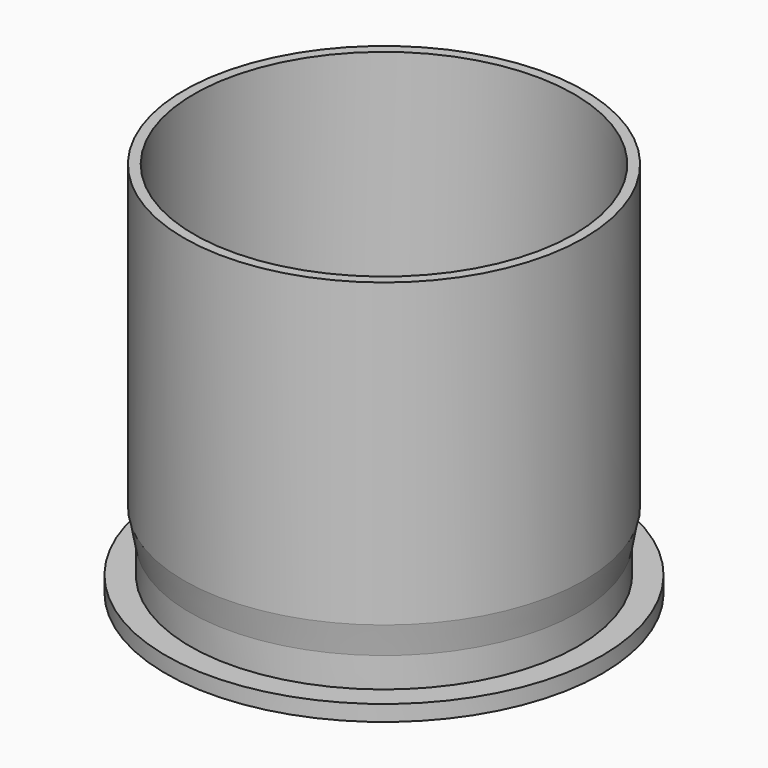
from build123d import *

# Parameters (mm, degrees)
F0_R     = 21.8313
F1_DEPTH = 1.5875
F2_R     = 19.3793862589
F3_DEPTH = 3
F4_R     = 19.4142729727
F5_DEPTH = 3
F5_TAPER = -10
F6_R     = 20
F7_DEPTH = 30.1498
F8_T     = 1
F10_D    = 12.7


# Not quite as in the source:
# - a length typed as a fraction of an inch, garbled in the dataset ("3 / 203.2 mm" for 3/8 in), is restored
# - a shell that OpenCascade refuses in one call is made with other operations: the cavity is built on its own and cut out


with BuildPart() as f1:
    # F0 (on Top) → F1 (new body)
    with BuildSketch(Plane.XY):
        Circle(F0_R)
    extrude(amount=F1_DEPTH)

    # F2 (on face) → F3 (join)
    with BuildSketch(Plane.XY.offset(1.5875)):
        Circle(F2_R)
    extrude(amount=F3_DEPTH)

    # F4 (on face) → F5 (join)
    with BuildSketch(Plane.XY.offset(4.5875)):
        Circle(F4_R)
    extrude(amount=F5_DEPTH, taper=F5_TAPER)

    # F6 (on face) → F7 (join)
    with BuildSketch(Plane.XY.offset(7.5875)):
        Circle(F6_R)
    extrude(amount=F7_DEPTH)

    # F8: shell of thickness 1, made by hand


with BuildPart() as f8_core1:
    # F8_t2: copy of F1
    add(f1.part)

    # the walls: a layer under each face that stays
    f8_faces = [f8_core1.faces().sort_by_distance(p)[0] for p in [
        (-20, 0, 22.6624),
        (17.5, -9.6296296296, 7.5875),
        (-19.6787634438, 0, 6.0875),
        (16.9874888511, -9.3476129128, 4.5875),
        (-19.3793862589, 0, 3.0875),
        (-14.5542, -14.5542, 1.5875),
        (-21.8313, 0, 0.79375),
        (0, 0, 0),
    ]]
    thicken(f8_faces, amount=-F8_T, mode=Mode.SUBTRACT)

    # F8_s3 → F8_t4 (revolve, cut)
    with BuildSketch(Plane.XZ):
        Polygon((19.9531019924, 7.5757635182), (19.9432539149, 8.5875), (19.1041542837, 8.5875), (18.9584461618, 7.7611481777), align=None)
    revolve(axis=Axis((0, 0, 7.5875), (0, 0, -1)), mode=Mode.SUBTRACT)

    # F8_s5 → F8_t6 (revolve, cut)
    with BuildSketch(Plane.XZ):
        Polygon((19.3893862589, 4.5775), (19.3793862589, 5.5875), (18.3793862589, 5.5875), (18.3793862589, 4.5875), align=None)
    revolve(axis=Axis((0, 0, 4.5875), (0, 0, 1)), mode=Mode.SUBTRACT)

    # F8_s7 → F8_t8 (revolve, cut)
    with BuildSketch(Plane.XZ):
        Polygon((19.3893862589, 1.5975), (18.3793862589, 1.5875), (18.3793862589, 0.5875), (19.3793862589, 0.5875), align=None)
    revolve(axis=Axis((0, 0, 1.5875), (0, 0, 1)), mode=Mode.SUBTRACT)


with BuildPart() as f1_1:
    add(f1.part)

    # what is left inside the walls is the cavity
    f8_cavity = [f8_core1.part.solids().sort_by_distance(p)[0] for p in [
        (-18.99, 0, 27.823804),
    ]]
    add(f8_cavity, mode=Mode.SUBTRACT)

    # F10 (through all)
    with Locations(Plane(origin=(0, 0, 0), x_dir=(1, 0, 0), z_dir=(0, 0, -1))):
        with Locations((0, 0)):
            Hole(F10_D / 2)


solid = f1_1.part
